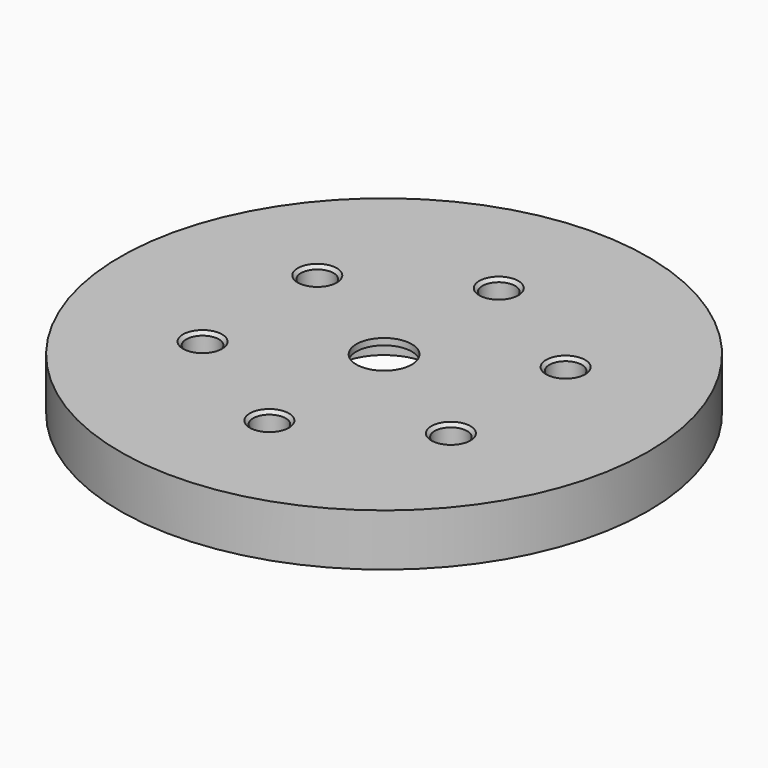
from build123d import *

# Parameters (mm, degrees)
F0_R           = 40.5
F1_DEPTH       = 8
F3_D           = 5
F3_CSINK_D     = 6
F3_CSINK_ANGLE = 90
F4_R           = 7.5
F5_DEPTH       = 7
F6_R           = 4.25
F7_DEPTH       = 1.001
F8_W           = 57
F8_H           = 57
F8_R           = 2.5
F8_R_2         = 7.5
F9_DEPTH       = 4
F10_R          = 5


# Not quite as in the source:
# - a feature names something its author has since deleted; it is built from what else it names


with BuildPart() as f1:
    # F0 (on Top) → F1 (new body)
    with BuildSketch(Plane.XY):
        Circle(F0_R)
    extrude(amount=F1_DEPTH)

    # F3 (through all)
    with Locations(Plane.XY.offset(8)):
        with Locations((0, 22), (19.0525588833, 11), (19.0525588833, -11), (0, -22), (-19.0525588833, -11), (-19.0525588833, 11)):
            CounterSinkHole(F3_D / 2, F3_CSINK_D / 2, counter_sink_angle=F3_CSINK_ANGLE)

    # F4 (on face) → F5 (cut)
    with BuildSketch(Plane(origin=(0, 0, 0), x_dir=(1, 0, 0), z_dir=(0, 0, -1))):
        Circle(F4_R)
    extrude(amount=-F5_DEPTH, mode=Mode.SUBTRACT)

    # F6 (on face) → F7 (cut, through all)
    with BuildSketch(Plane(origin=(0, 0, 7), x_dir=(1, 0, 0), z_dir=(0, 0, -1))):
        Circle(F6_R)
    extrude(amount=-F7_DEPTH, mode=Mode.SUBTRACT)

    # F8 (on face) → F9 (cut)
    with BuildSketch(Plane(origin=(0, 0, 0), x_dir=(1, 0, 0), z_dir=(0, 0, -1))):
        Rectangle(F8_W, F8_H)
        with Locations((-19.0525588833, -11)):
            Circle(F8_R, mode=Mode.SUBTRACT)
        with Locations((0, -22)):
            Circle(F8_R, mode=Mode.SUBTRACT)
        with Locations((19.0525588833, -11)):
            Circle(F8_R, mode=Mode.SUBTRACT)
        with Locations((-19.0525588833, 11)):
            Circle(F8_R, mode=Mode.SUBTRACT)
        Circle(F8_R_2, mode=Mode.SUBTRACT)
        with Locations((19.0525588833, 11)):
            Circle(F8_R, mode=Mode.SUBTRACT)
        with Locations((0, 22)):
            Circle(F8_R, mode=Mode.SUBTRACT)
    extrude(amount=-F9_DEPTH, mode=Mode.SUBTRACT)

    # F10
    f10_edges = [f1.edges().sort_by_distance(p)[0] for p in [
        (28.5, 28.5, 2),
        (28.5, -28.5, 2),
        (-28.5, -28.5, 2),
        (-28.5, 28.5, 2),
    ]]
    fillet(f10_edges, radius=F10_R)


solid = f1.part
